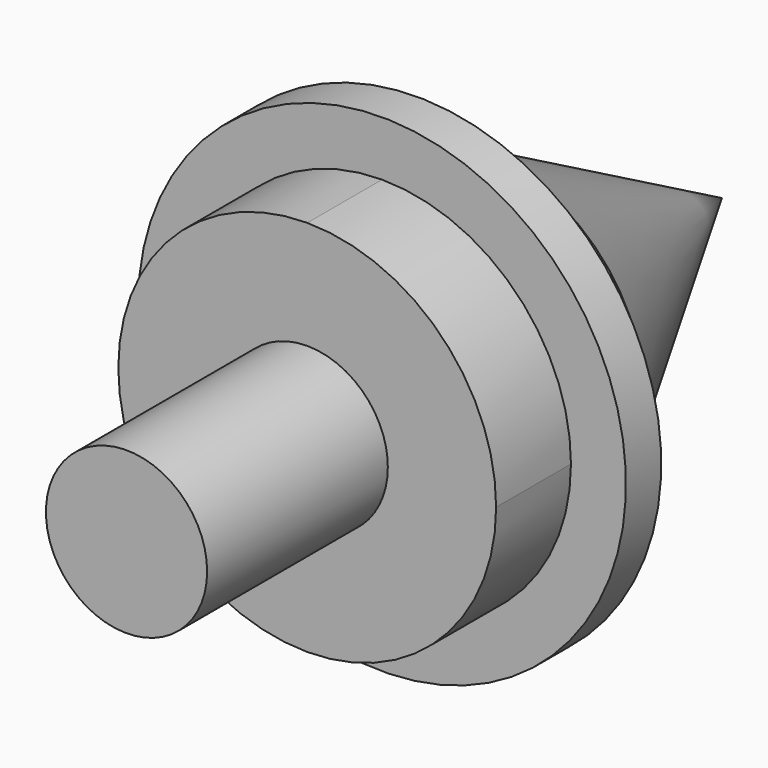
from build123d import *

# Parameters (mm, degrees)
F2_R     = 10.9427513267
F6_DEPTH = 12.7


# Not quite as in the source:
# - a feature of the source that left no trace in its solid (it failed there, or was rolled back) is left out


with BuildPart() as f1:
    # F0 (on Top) → F1 (revolve)
    with BuildSketch(Plane.XY):
        Polygon((-22.4952585995, 7.654638961), (-22.4952585995, 0), (0, 0), (0, 51.6905076802), (-22.4952585995, 10.4665467516), (-5.6238141842, 10.4665467516), (-5.6238141842, 7.654638961), align=None)
        Polygon((-22.4952585995, 0), (-33.1180207431, 0), (-33.1180207431, -5.9848567471), (0, -5.9848567471), (0, 0), align=None)
    revolve(axis=Axis((0, -2.9924283735, 0), (0, -1, 0)))

    # F4: sweep along a path in F3
    with BuildLine(Plane.XY) as f4_path:
        Line((0, -6.7567974329), (0, -50.1213520765))
    # F2 (on face) → F4 (sweep)
    with BuildSketch(Plane.XZ.offset(5.9848567471)):
        Circle(F2_R)
    sweep(path=f4_path.line)

    # F5 (on face) → F6 (join)
    with BuildSketch(Plane.XZ.offset(5.9848567471)):
        with BuildLine():
            ThreePointArc((0, 25.6462656645), (-18.1346483635, -18.1346483635), (25.6462656645, 0))
            ThreePointArc((25.6462656645, 0), (18.1346483635, 18.1346483635), (0, 25.6462656645))
        make_face()
        with BuildLine():
            ThreePointArc((-10.2304533567, 3.8835075273), (-6.214802871, 9.0066659687), (0, 10.9427513267))
            ThreePointArc((0, 10.9427513267), (6.3686758751, 8.8985265182), (10.3578760896, 3.5296188901))
            ThreePointArc((10.3578760896, 3.5296188901), (10.7955423421, 1.7888745451), (10.9427513267, 0))
            ThreePointArc((10.9427513267, 0), (9.4510721789, -5.5155272882), (5.3827161292, -9.5273382259))
            ThreePointArc((5.3827161292, -9.5273382259), (0, -10.9427513267), (-5.3827161292, -9.5273382259))
            ThreePointArc((-5.3827161292, -9.5273382259), (-10.2910379118, -3.7199926472), (-10.2304533567, 3.8835075273))
        make_face(mode=Mode.SUBTRACT)
    extrude(amount=F6_DEPTH)


solid = f1.part
